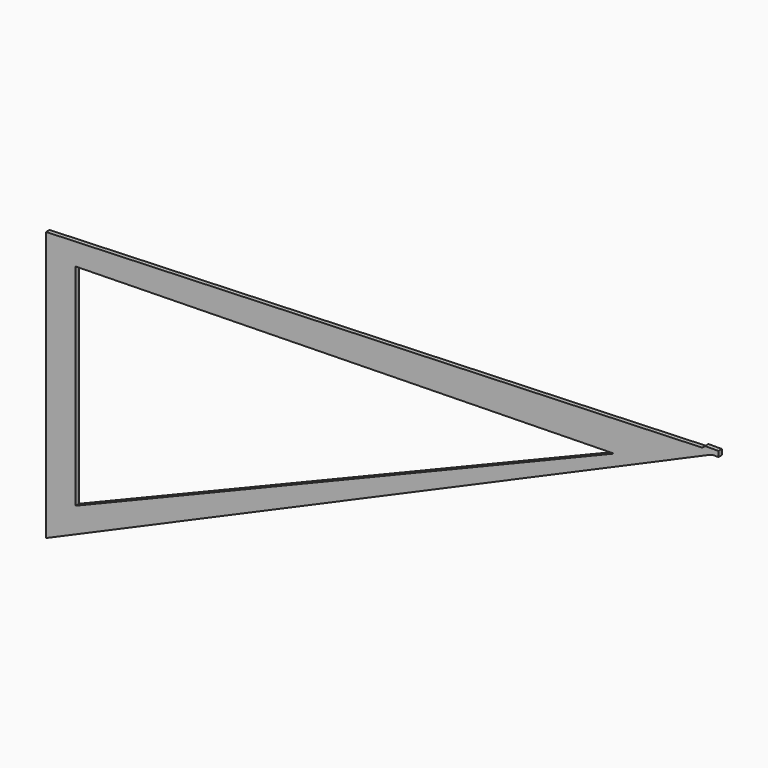
from build123d import *

# Parameters (mm, degrees)
F1_DEPTH    = 2
F2_DEPTH    = 2
F3_DEPTH    = 2
F4_DEPTH    = 2
F5_T1_DEPTH = 4
F6_R        = 6.5


# Not quite as in the source:
# - a fillet or chamfer that OpenCascade refuses, or shapes differently, is made with other operations: its cross-section is extruded or revolved along the edge and cut away or added


with BuildPart() as f1:
    # F0 (on Front) → F1 (new body)
    with BuildSketch(Plane.XZ):
        Polygon((611.2015247345, 21.8497800332), (0, 0), (0, -250), (617.4515247345, 18.9482106362), (611.2015247345, 18.9482106362), align=None)
        Polygon((27.5068562478, -214.647129178), (27.5068562478, -19.3058601132), (526.7680287361, -9.7110727802), align=None, mode=Mode.SUBTRACT)
    extrude(amount=F1_DEPTH)

    # F0 (on Front) → F2 (join)
    with BuildSketch(Plane.XZ):
        Polygon((611.2015247345, 21.8497800332), (0, 0), (0, -250), (617.4515247345, 18.9482106362), (611.2015247345, 18.9482106362), align=None)
        Polygon((27.5068562478, -214.647129178), (27.5068562478, -19.3058601132), (526.7680287361, -9.7110727802), align=None, mode=Mode.SUBTRACT)
    extrude(amount=-F2_DEPTH)

    # F0 (on Front) → F3 (join)
    with BuildSketch(Plane.XZ):
        Polygon((611.2015247345, 23.9482106362), (611.2015247345, 21.8497800332), (611.2015247345, 18.9482106362), (617.4515247345, 18.9482106362), (623.7015247345, 18.9482106362), (623.7015247345, 23.9482106362), align=None)
    extrude(amount=F3_DEPTH)

    # F0 (on Front) → F4 (join)
    with BuildSketch(Plane.XZ):
        Polygon((611.2015247345, 23.9482106362), (611.2015247345, 21.8497800332), (611.2015247345, 18.9482106362), (617.4515247345, 18.9482106362), (623.7015247345, 18.9482106362), (623.7015247345, 23.9482106362), align=None)
    extrude(amount=-F4_DEPTH)

    # F5: fillet of radius 5 on 1 edges, made by hand

    # F5_s2 → F5_t1 (join)
    with BuildSketch(Plane.XZ.offset(-2)):
        with BuildLine():
            ThreePointArc((611.2015247345, 23.9482106362), (609.476442407, 22.3435494733), (607.20803479, 21.7070171746))
            Line((607.20803479, 21.7070171746), (611.2015247345, 21.8497800332))
            Line((611.2015247345, 21.8497800332), (611.2015247345, 23.9482106362))
        make_face()
    extrude(amount=F5_T1_DEPTH)

    # F6
    f6_edges = [f1.edges().sort_by_distance(p)[0] for p in [
        (617.451525, 0, 18.948211),
    ]]
    fillet(f6_edges, radius=F6_R)


solid = f1.part
